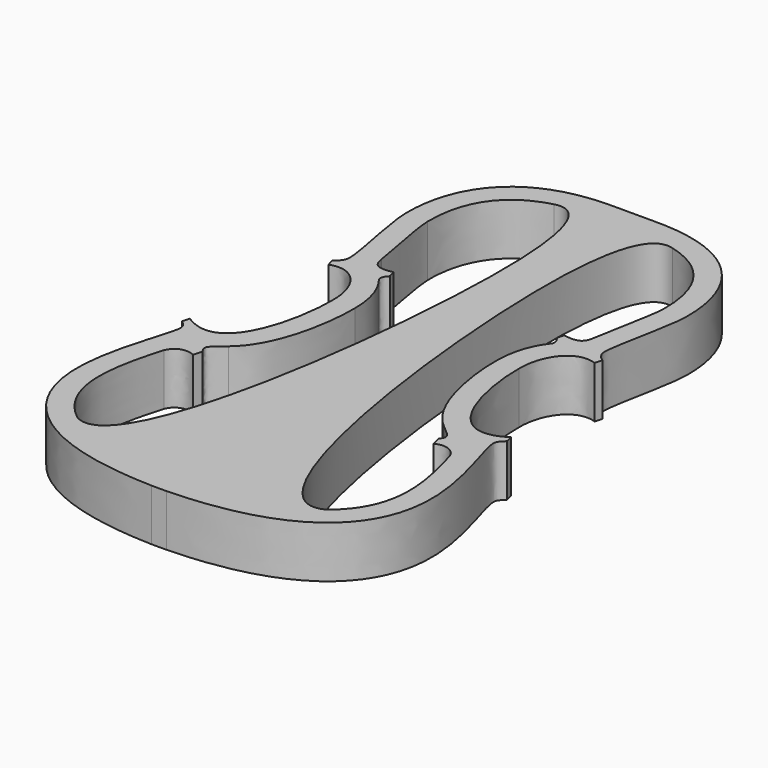
from build123d import *

# Parameters (mm, degrees)
F1_DEPTH = 35
F4_DEPTH = 35.0010001
F7_W     = 17
F7_H     = 12.264450103
F8_DEPTH = 30


# Not quite as in the source:
# - ends of sketch curves that miss each other by under 0.0002 mm in the source are joined
# - the dataset's text gives a spline's control points without its knots; the knots are read off the source's solid


with BuildPart() as f1:
    # F0 (on Top) → F1 (new body)
    with BuildSketch(Plane.XY):
        with BuildLine():
            ThreePointArc((7.5, 284.7219171226), (5.3033008589, 290.0252179815), (0, 292.2219171226))
            Line((0, 292.2219171226), (-1, 292.2219171226))
            Line((-1, 292.2219171226), (-1, -119.7780828774))
            Line((-1, -119.7780828774), (4, -119.7780828774))
            add(Edge.make_bspline(
                [(109, 37.3938740408), (105.6307440999, 34.3802133174), (101.4956652983, 29.6953939154), (138.6392780904, -56.2531371267), (89.0329927206, -117.4921383262), (4, -119.7780828774)],
                knots=[0, 0, 0, 0, 0.1283809688, 0.4939795161, 1, 1, 1, 1], degree=3))
            Line((109, 37.3938740408), (107.7, 42.2219171226))
            add(Edge.make_bspline(
                [(62, 106.2219171226), (61.3599307835, 81.0817395672), (72.3934512258, 19.5276373401), (107.7, 42.2219171226)],
                knots=[0, 0, 0, 0, 78.6415284694, 78.6415284694, 78.6415284694, 78.6415284694], degree=3))
            add(Edge.make_bspline(
                [(89.1, 136.4219171226), (73.1859058142, 141.8396075591), (61.6909898818, 125.2358471378), (62, 106.2219171226)],
                knots=[0, 0, 0, 0, 40.5764710146, 40.5764710146, 40.5764710146, 40.5764710146], degree=3))
            Line((89.1, 136.4219171226), (90.5, 141.2219171226))
            add(Edge.make_bspline(
                [(94, 207.2219171226), (93.7038545596, 193.8460895116), (83.3685824993, 151.8432754504), (85.6278354948, 144.9055942149), (90.5, 141.2219171226)],
                knots=[0, 0, 0, 0, 0.6721964469, 1, 1, 1, 1], degree=3))
            add(Edge.make_bspline(
                [(94, 207.2219171226), (94.8413443307, 245.2224236083), (74.4074434042, 283.3588123322), (12.5, 282.7219171226)],
                knots=[0, 0, 0, 0, 111.0968046345, 111.0968046345, 111.0968046345, 111.0968046345], degree=3))
            Line((12.5, 282.7219171226), (7.5, 282.7219171226))
            Line((7.5, 282.7219171226), (7.5, 284.7219171226))
        make_face()
    extrude(amount=F1_DEPTH)

    # F2 (on face) → F4 (cut, through all)
    with BuildSketch(Plane.XY.offset(35)):
        with BuildLine():
            add(Edge.make_bspline(
                [(39, 264.8111790782), (18.2084372354, 270.6442923223), (1.2745943331, 165.1183841916), (43.5392409562, -105.3502410651), (83.406358512, -83.4033276804)],
                knots=[0, 0, 0, 0, 0.3896638766, 1, 1, 1, 1], degree=3))
            add(Edge.make_bspline(
                [(83.406358512, -83.4033276804), (85.1174112218, -82.0661920108), (88.3462816429, -79.2479991923), (92.4386290016, -74.7800356068), (95.8678975083, -70.0247382255), (98.6429146246, -65.0437340993), (100.8205672733, -59.8159067277), (102.4360343795, -54.3254230325), (103.3298022671, -49.5289794375), (103.778869156, -45.5660462029), (103.9839616301, -42.534437951), (104.0582272293, -39.4464470468), (104.0064715057, -36.2769195828), (103.8350865018, -33.0466394449), (103.4569657427, -28.6754381448), (102.7243882007, -23.1282672783), (101.5051996885, -16.4505011137), (100.0303086017, -9.857805046), (98.3885088389, -3.4487796992), (96.9749622962, 1.5996216644), (96.1391197573, 4.4769668588), (95.8745243685, 5.3809508195)],
                knots=[0.2515767455, 0.2515767455, 0.2515767455, 0.2515767455, 0.28125, 0.3125, 0.34375, 0.375, 0.40625, 0.4375, 0.46875, 0.484375, 0.5, 0.515625, 0.53125, 0.546875, 0.5625, 0.59375, 0.625, 0.65625, 0.6875, 0.71875, 0.733386008, 0.733386008, 0.733386008, 0.733386008], degree=3))
            add(Edge.make_bspline(
                [(80.483276842, 10.9469161382), (87.2777308402, 14.1946932067), (93.4604853391, 11.2472865732), (95.8745243685, 5.3809508195)],
                knots=[0, 0, 0, 0, 16.3667496892, 16.3667496892, 16.3667496892, 16.3667496892], degree=3))
            Line((80.483276842, 10.9469161382), (78.8500127218, 17.0126619354))
            add(Edge.make_bspline(
                [(78.8500127218, 17.0126619354), (83.590825933, 22.6212095236), (78.5805061459, 23.9398982376), (71.9697522905, 30.2162654084)],
                knots=[0, 0, 0, 0, 14.8886912882, 14.8886912882, 14.8886912882, 14.8886912882], degree=3))
            add(Edge.make_bspline(
                [(71.9697522905, 30.2162654084), (71.8480545471, 30.3172897241), (70.6395337945, 31.3329639362), (68.4978847961, 33.3673908409), (64.9083916723, 37.4880347031), (61.176393476, 43.0179757376), (57.5864656351, 50.0588191493), (54.6822609486, 57.3907351829), (52.3392454886, 64.9035625481), (50.4783482148, 72.4783616859), (49.0459112886, 79.9856884701), (48.0028968526, 87.2901461757), (47.319327939, 94.2563139822), (46.9788520113, 100.6423943553), (46.9578896974, 104.5062338542), (46.9976044777, 106.2988976338)],
                knots=[0.3090268116, 0.3090268116, 0.3090268116, 0.3090268116, 0.3125, 0.34375, 0.375, 0.4375, 0.5, 0.5625, 0.625, 0.6875, 0.75, 0.8125, 0.875, 0.9375, 0.9966391535, 0.9966391535, 0.9966391535, 0.9966391535], degree=3))
            add(Edge.make_bspline(
                [(46.9976044777, 106.2988976338), (46.9641100842, 109.3389993919), (47.357470233, 115.4439738443), (49.3024122501, 124.2512445301), (52.1119143651, 131.2090770511), (55.022387203, 136.2126140487), (56.662649951, 138.4911897815), (57.4729083813, 139.5079689731)],
                knots=[0.0042445232, 0.0042445232, 0.0042445232, 0.0042445232, 0.125, 0.25, 0.375, 0.4375, 0.4908706686, 0.4908706686, 0.4908706686, 0.4908706686], degree=3))
            add(Edge.make_bspline(
                [(55.5, 146.2219171226), (57.2690921243, 144.6406759419), (59.0109937029, 141.6761428289), (57.4729083813, 139.5079689731)],
                knots=[0, 0, 0, 0, 6.9978344121, 6.9978344121, 6.9978344121, 6.9978344121], degree=3))
            Line((55.5, 146.2219171226), (56.9, 151.0219171226))
            add(Edge.make_bspline(
                [(56.9, 151.0219171226), (68.3496427976, 148.7567939734), (70.0243914902, 152.8649312806), (71.0326328697, 158.4451697773)],
                knots=[0, 0, 0, 0, 15.9635833009, 15.9635833009, 15.9635833009, 15.9635833009], degree=3))
            add(Edge.make_bspline(
                [(71.0326328697, 158.4451697773), (71.1247616786, 159.100226934), (71.3393545708, 160.548355676), (71.7125660649, 162.8656604268), (72.1467629093, 165.3983350302), (72.7721347144, 168.8906596969), (73.6237749338, 173.4433587258), (74.7013069468, 179.087073127), (75.7764109904, 184.7720975313), (76.7899048927, 190.346659005), (77.6817019844, 195.6455230688), (78.3918616247, 200.482818984), (78.7837087545, 203.9456863865), (78.9559633752, 206.2191138107), (78.9947689636, 207.151682209), (79.0036751106, 207.5539409322)],
                knots=[0.3796250563, 0.3796250563, 0.3796250563, 0.3796250563, 0.40625, 0.4375, 0.46875, 0.5, 0.5625, 0.625, 0.6875, 0.75, 0.8125, 0.875, 0.9375, 0.96875, 1, 1, 1, 1], degree=3))
            add(Edge.make_bspline(
                [(79.0036751106, 207.5539409322), (79.0933577763, 211.6045853551), (78.701590995, 219.6244916849), (76.7053840536, 229.0121846533), (74.1906772139, 235.9357295448), (71.8428042818, 240.8038728478), (69.0226174243, 245.3280447727), (65.7053447856, 249.5028714335), (61.8450593279, 253.3297536944), (57.3725777247, 256.8064047755), (52.2003401223, 259.915179624), (46.233410561, 262.6157044954), (41.5966583515, 264.1240071717), (39.0739544407, 264.7917281117), (39, 264.8111790782)],
                knots=[0, 0, 0, 0, 0.125, 0.25, 0.3125, 0.375, 0.4375, 0.5, 0.5625, 0.625, 0.6875, 0.75, 0.8125, 0.8143837178, 0.8143837178, 0.8143837178, 0.8143837178], degree=3))
        make_face()
    extrude(amount=-F4_DEPTH, mode=Mode.SUBTRACT)

    # F6: F1 across face


with BuildPart() as f1_1:
    add(f1.part)
    add(f1.part.mirror(Plane(origin=(-1, 86.2219171226, 17.5), x_dir=(0, -1, 0), z_dir=(-1, 0, 0))))

    # F7 (on face) → F8 (cut)
    with BuildSketch(Plane.XY.offset(35)):
        with Locations((-1, 288.8541421741)):
            Rectangle(F7_W, F7_H)
    extrude(amount=-F8_DEPTH, mode=Mode.SUBTRACT)


solid = f1_1.part
